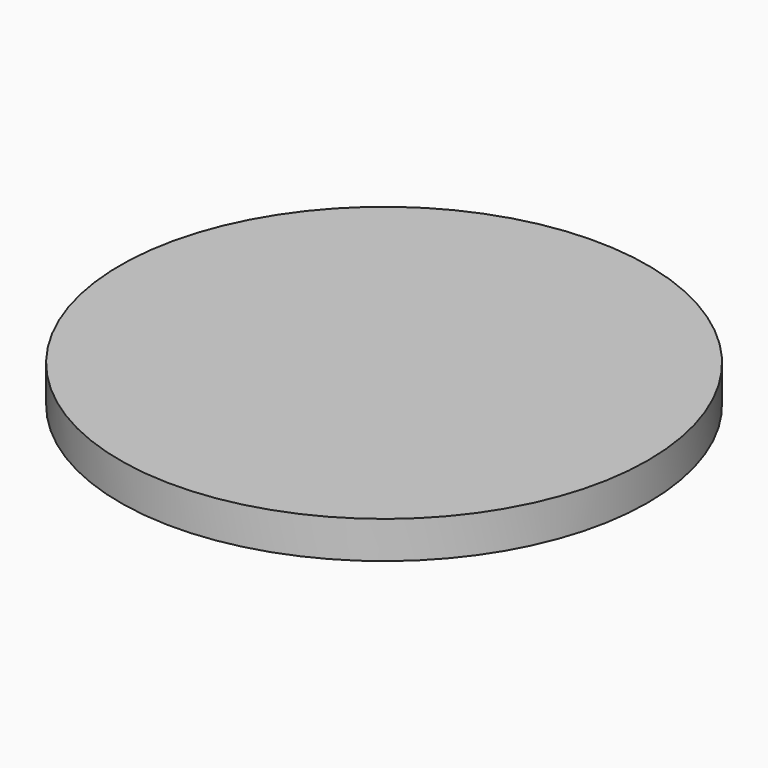
from build123d import *

# Parameters (mm, degrees)
F2_R     = 35.5
F3_DEPTH = 5


# Not quite as in the source:
# - the program builds the solid bodies; features that only make, move or delete a surface that nothing else refers to are left out


with BuildPart() as f3:
    # F2 (on Top) → F3 (new body)
    with BuildSketch(Plane.XY):
        with Locations((-46.3043488562, 17.1195659786)):
            Circle(F2_R)
    extrude(amount=F3_DEPTH)


solid = f3.part
